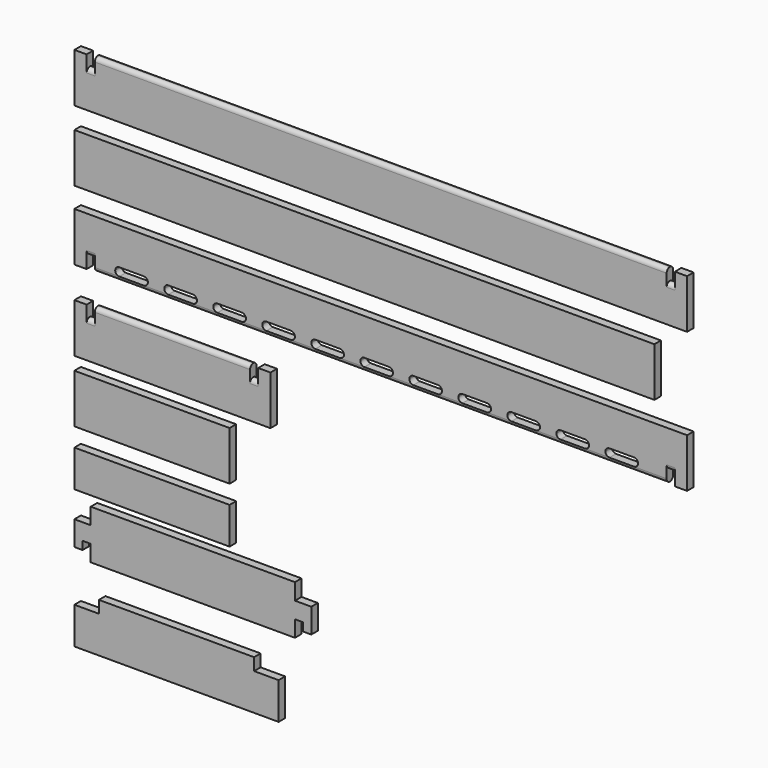
from build123d import *

# Parameters (mm, degrees)
F0_W     = 476.25
F0_H     = 38.1
F2_DEPTH = 6.35
F1_W     = 152.4
F1_H     = 38.1
F1_W_2   = 120.65
F1_H_2   = 28.575
F1_W_3   = 184.15
F1_W_4   = 158.75
F3_W     = 476.25
F3_H     = 38.1
F4_DEPTH = 6.35
F5_W     = 6.35
F5_H     = 9.525
F5_W_2   = 12.7
F5_H_2   = 12.7
F5_W_3   = 19.05
F6_DEPTH = 6.35
F7_R     = 3.17499
F7_2_R   = 3.17499
F7_3_R   = 3.17499
F8_W     = 450.85
F8_H     = 38.1
F9_DEPTH = 6.35


# Not quite as in the source:
# - a fillet or chamfer is up to 0.001 mm smaller than in the source, because OpenCascade refuses the exact size
# - a feature names something its author has since deleted; it is built from what else it names


with BuildPart() as f2:
    # F0 (on Front) → F2 (new body)
    with BuildSketch(Plane.XZ):
        with Locations((238.125, 19.05)):
            Rectangle(F0_W, F0_H)
    extrude(amount=-F2_DEPTH)


with BuildPart() as f2b:
    # F1 (on Front) → F2, piece 2 (new body)
    with BuildSketch(Plane.XZ):
        with Locations((76.2, -152.1868369205)):
            Rectangle(F1_W, F1_H)
    extrude(amount=-F2_DEPTH)


with BuildPart() as f2c:
    # F1 (on Front) → F2, piece 3 (new body)
    with BuildSketch(Plane.XZ):
        with Locations((60.325, -200.4974952459)):
            Rectangle(F1_W_2, F1_H)
    extrude(amount=-F2_DEPTH)


with BuildPart() as f2d:
    # F1 (on Front) → F2, piece 4 (new body)
    with BuildSketch(Plane.XZ):
        with Locations((60.325, -248.3239487648)):
            Rectangle(F1_W_2, F1_H_2)
    extrude(amount=-F2_DEPTH)


with BuildPart() as f2e:
    # F1 (on Front) → F2, piece 5 (new body)
    with BuildSketch(Plane.XZ):
        with Locations((92.075, -289.424034071)):
            Rectangle(F1_W_3, F1_H)
    extrude(amount=-F2_DEPTH)


with BuildPart() as f2f:
    # F1 (on Front) → F2, piece 6 (new body)
    with BuildSketch(Plane.XZ):
        with Locations((79.375, -351.1140069485)):
            Rectangle(F1_W_4, F1_H)
    extrude(amount=-F2_DEPTH)


with BuildPart() as f4:
    # F3 (on Front) → F4 (new body)
    with BuildSketch(Plane.XZ):
        with Locations((238.125, -89.7808095932)):
            Rectangle(F3_W, F3_H)
    extrude(amount=-F4_DEPTH)


with BuildPart() as f6_tool:
    # F5 (on Front) → F6 (new body, through all)
    with BuildSketch(Plane.XZ):
        with Locations((12.7, 33.3375)):
            Rectangle(F5_W, F5_H)
        with Locations((463.55, 33.3375)):
            Rectangle(F5_W, F5_H)
        with Locations((12.7, -104.0683095932)):
            Rectangle(F5_W, F5_H)
        with Locations((463.55, -104.0683095932)):
            Rectangle(F5_W, F5_H)
        with Locations((12.7, -137.8993369205)):
            Rectangle(F5_W, F5_H)
        with Locations((139.7, -137.8993369205)):
            Rectangle(F5_W, F5_H)
        with BuildLine():
            Line((53.975, -99.3058095932), (34.925, -99.3058095932))
            ThreePointArc((34.925, -99.3058095932), (32.6799359697, -100.2357455629), (31.75, -102.4808095932))
            ThreePointArc((31.75, -102.4808095932), (32.6799359697, -104.7258736235), (34.925, -105.6558095932))
            Line((34.925, -105.6558095932), (53.975, -105.6558095932))
            ThreePointArc((53.975, -105.6558095932), (56.2200640303, -104.7258736235), (57.15, -102.4808095932))
            ThreePointArc((57.15, -102.4808095932), (56.2200640303, -100.2357455629), (53.975, -99.3058095932))
        make_face()
        with BuildLine():
            Line((92.075, -99.3058095932), (73.025, -99.3058095932))
            ThreePointArc((73.025, -99.3058095932), (70.7799359697, -100.2357455629), (69.85, -102.4808095932))
            ThreePointArc((69.85, -102.4808095932), (70.7799359697, -104.7258736235), (73.025, -105.6558095932))
            Line((73.025, -105.6558095932), (92.075, -105.6558095932))
            ThreePointArc((92.075, -105.6558095932), (94.3200640303, -104.7258736235), (95.25, -102.4808095932))
            ThreePointArc((95.25, -102.4808095932), (94.3200640303, -100.2357455629), (92.075, -99.3058095932))
        make_face()
        with BuildLine():
            Line((130.175, -99.3058095932), (111.125, -99.3058095932))
            ThreePointArc((111.125, -99.3058095932), (108.8799359697, -100.2357455629), (107.95, -102.4808095932))
            ThreePointArc((107.95, -102.4808095932), (108.8799359697, -104.7258736235), (111.125, -105.6558095932))
            Line((111.125, -105.6558095932), (130.175, -105.6558095932))
            ThreePointArc((130.175, -105.6558095932), (132.4200640303, -104.7258736235), (133.35, -102.4808095932))
            ThreePointArc((133.35, -102.4808095932), (132.4200640303, -100.2357455629), (130.175, -99.3058095932))
        make_face()
        with BuildLine():
            Line((168.275, -99.3058095932), (149.225, -99.3058095932))
            ThreePointArc((149.225, -99.3058095932), (146.9799359697, -100.2357455629), (146.05, -102.4808095932))
            ThreePointArc((146.05, -102.4808095932), (146.9799359697, -104.7258736235), (149.225, -105.6558095932))
            Line((149.225, -105.6558095932), (168.275, -105.6558095932))
            ThreePointArc((168.275, -105.6558095932), (170.5200640303, -104.7258736235), (171.45, -102.4808095932))
            ThreePointArc((171.45, -102.4808095932), (170.5200640303, -100.2357455629), (168.275, -99.3058095932))
        make_face()
        with BuildLine():
            Line((206.375, -99.3058095932), (187.325, -99.3058095932))
            ThreePointArc((187.325, -99.3058095932), (185.0799359697, -100.2357455629), (184.15, -102.4808095932))
            ThreePointArc((184.15, -102.4808095932), (185.0799359697, -104.7258736235), (187.325, -105.6558095932))
            Line((187.325, -105.6558095932), (206.375, -105.6558095932))
            ThreePointArc((206.375, -105.6558095932), (208.6200640303, -104.7258736235), (209.55, -102.4808095932))
            ThreePointArc((209.55, -102.4808095932), (208.6200640303, -100.2357455629), (206.375, -99.3058095932))
        make_face()
        with BuildLine():
            Line((244.475, -99.3058095932), (225.425, -99.3058095932))
            ThreePointArc((225.425, -99.3058095932), (223.1799359697, -100.2357455629), (222.25, -102.4808095932))
            ThreePointArc((222.25, -102.4808095932), (223.1799359697, -104.7258736235), (225.425, -105.6558095932))
            Line((225.425, -105.6558095932), (244.475, -105.6558095932))
            ThreePointArc((244.475, -105.6558095932), (246.7200640303, -104.7258736235), (247.65, -102.4808095932))
            ThreePointArc((247.65, -102.4808095932), (246.7200640303, -100.2357455629), (244.475, -99.3058095932))
        make_face()
        with BuildLine():
            Line((282.575, -99.3058095932), (263.525, -99.3058095932))
            ThreePointArc((263.525, -99.3058095932), (261.2799359697, -100.2357455629), (260.35, -102.4808095932))
            ThreePointArc((260.35, -102.4808095932), (261.2799359697, -104.7258736235), (263.525, -105.6558095932))
            Line((263.525, -105.6558095932), (282.575, -105.6558095932))
            ThreePointArc((282.575, -105.6558095932), (284.8200640303, -104.7258736235), (285.75, -102.4808095932))
            ThreePointArc((285.75, -102.4808095932), (284.8200640303, -100.2357455629), (282.575, -99.3058095932))
        make_face()
        with BuildLine():
            Line((320.675, -99.3058095932), (301.625, -99.3058095932))
            ThreePointArc((301.625, -99.3058095932), (299.3799359697, -100.2357455629), (298.45, -102.4808095932))
            ThreePointArc((298.45, -102.4808095932), (299.3799359697, -104.7258736235), (301.625, -105.6558095932))
            Line((301.625, -105.6558095932), (320.675, -105.6558095932))
            ThreePointArc((320.675, -105.6558095932), (322.9200640303, -104.7258736235), (323.85, -102.4808095932))
            ThreePointArc((323.85, -102.4808095932), (322.9200640303, -100.2357455629), (320.675, -99.3058095932))
        make_face()
        with BuildLine():
            Line((358.775, -99.3058095932), (339.725, -99.3058095932))
            ThreePointArc((339.725, -99.3058095932), (337.4799359697, -100.2357455629), (336.55, -102.4808095932))
            ThreePointArc((336.55, -102.4808095932), (337.4799359697, -104.7258736235), (339.725, -105.6558095932))
            Line((339.725, -105.6558095932), (358.775, -105.6558095932))
            ThreePointArc((358.775, -105.6558095932), (361.0200640303, -104.7258736235), (361.95, -102.4808095932))
            ThreePointArc((361.95, -102.4808095932), (361.0200640303, -100.2357455629), (358.775, -99.3058095932))
        make_face()
        with BuildLine():
            Line((396.875, -99.3058095932), (377.825, -99.3058095932))
            ThreePointArc((377.825, -99.3058095932), (375.5799359697, -100.2357455629), (374.65, -102.4808095932))
            ThreePointArc((374.65, -102.4808095932), (375.5799359697, -104.7258736235), (377.825, -105.6558095932))
            Line((377.825, -105.6558095932), (396.875, -105.6558095932))
            ThreePointArc((396.875, -105.6558095932), (399.1200640303, -104.7258736235), (400.05, -102.4808095932))
            ThreePointArc((400.05, -102.4808095932), (399.1200640303, -100.2357455629), (396.875, -99.3058095932))
        make_face()
        with Locations((6.35, -276.724034071)):
            Rectangle(F5_W_2, F5_H_2)
        with Locations((177.8, -276.724034071)):
            Rectangle(F5_W_2, F5_H_2)
        Polygon((177.8, -295.774034071), (171.45, -295.774034071), (171.45, -308.474034071), (184.15, -308.474034071), (184.15, -302.124034071), (177.8, -302.124034071), align=None)
        Polygon((12.7, -295.774034071), (6.35, -295.774034071), (6.35, -302.124034071), (0, -302.124034071), (0, -308.474034071), (12.7, -308.474034071), align=None)
        with Locations((9.525, -336.8265069485)):
            Rectangle(F5_W_3, F5_H)
        with Locations((149.225, -336.8265069485)):
            Rectangle(F5_W_3, F5_H)
        with BuildLine():
            Line((434.975, -99.3058095932), (415.925, -99.3058095932))
            ThreePointArc((415.925, -99.3058095932), (413.6799359697, -100.2357455629), (412.75, -102.4808095932))
            ThreePointArc((412.75, -102.4808095932), (413.6799359697, -104.7258736235), (415.925, -105.6558095932))
            Line((415.925, -105.6558095932), (434.975, -105.6558095932))
            ThreePointArc((434.975, -105.6558095932), (437.2200640303, -104.7258736235), (438.15, -102.4808095932))
            ThreePointArc((438.15, -102.4808095932), (437.2200640303, -100.2357455629), (434.975, -99.3058095932))
        make_face()
    extrude(amount=-F6_DEPTH)


with BuildPart() as f2_1:
    add(f2.part)

    # F6: cut by f6_tool
    add(f6_tool.part, mode=Mode.SUBTRACT)

    # F7 (radius 3.175 in the source; OpenCascade refuses exactly that, so slightly less here)
    f7_edges = [f2_1.edges().sort_by_distance(p)[0] for p in [
        (238.125, 0, 38.1),
        (238.125, 6.35, 38.1),
        (12.7, 0, 28.575),
        (12.7, 6.35, 28.575),
        (463.55, 6.35, 28.575),
        (463.55, 0, 28.575),
    ]]
    fillet(f7_edges, radius=F7_R)


with BuildPart() as f2b_1:
    add(f2b.part)

    # F6: cut by f6_tool
    add(f6_tool.part, mode=Mode.SUBTRACT)

    # F7#2 (radius 3.175 in the source; OpenCascade refuses exactly that, so slightly less here)
    f7_2_edges = [f2b_1.edges().sort_by_distance(p)[0] for p in [
        (76.2, 6.35, -133.136837),
        (76.2, 0, -133.136837),
        (12.7, 6.35, -142.661837),
        (139.7, 0, -142.661837),
        (139.7, 6.35, -142.661837),
        (12.7, 0, -142.661837),
    ]]
    fillet(f7_2_edges, radius=F7_2_R)


with BuildPart() as f2e_1:
    add(f2e.part)

    # F6: cut by f6_tool
    add(f6_tool.part, mode=Mode.SUBTRACT)


with BuildPart() as f2f_1:
    add(f2f.part)

    # F6: cut by f6_tool
    add(f6_tool.part, mode=Mode.SUBTRACT)


with BuildPart() as f4_1:
    add(f4.part)

    # F6: cut by f6_tool
    add(f6_tool.part, mode=Mode.SUBTRACT)

    # F7#3 (radius 3.175 in the source; OpenCascade refuses exactly that, so slightly less here)
    f7_3_edges = [f4_1.edges().sort_by_distance(p)[0] for p in [
        (238.125, 0, -108.83081),
        (238.125, 6.35, -108.83081),
        (12.7, 6.35, -99.30581),
        (12.7, 0, -99.30581),
        (463.55, 0, -99.30581),
        (463.55, 6.35, -99.30581),
    ]]
    fillet(f7_3_edges, radius=F7_3_R)


with BuildPart() as f9:
    # F8 (on Front) → F9 (new body)
    with BuildSketch(Plane.XZ):
        with Locations((225.425, -35.7729031265)):
            Rectangle(F8_W, F8_H)
    extrude(amount=-F9_DEPTH)


solid = Compound([f2c.part, f2d.part, f2_1.part, f2b_1.part, f2e_1.part, f2f_1.part, f4_1.part, f9.part])
